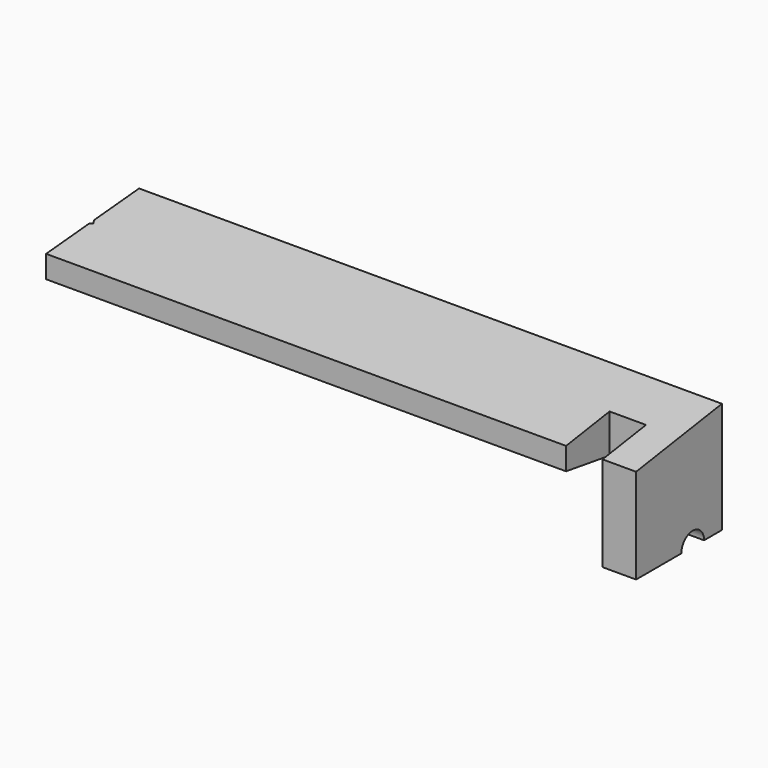
from build123d import *

# Parameters (mm, degrees)
F5_DEPTH  = 69.9135
F7_DEPTH  = 3.98018
F9_DEPTH  = 3.26644
F10_W     = 4.318
F10_H     = 6.4389
F11_DEPTH = 25.4
F12_R     = 1.68275
F13_DEPTH = 69.9145
F16_DEPTH = 13.17344
F18_DEPTH = 13.17344


# Not quite as in the source:
# - a variable given as a bare number and used for a length is read in inches; the dataset says mm whatever the document's units were


with BuildPart() as f5:
    # F4 (on Right) → F5 (new body)
    with BuildSketch(Plane.YZ):
        Polygon((12.7127, 13.17244), (0, 11.24458), (0, 8.59028), (12.7127, 6.66242), align=None)
    extrude(amount=-F5_DEPTH)

    # F6 (on face) → F7 (join)
    with BuildSketch(Plane.YZ):
        Polygon((12.7127, 0), (12.7127, 6.66242), (0, 8.59028), (0, 0), align=None)
    extrude(amount=-F7_DEPTH)

    # F8 (on face) → F9 (join)
    with BuildSketch(Plane(origin=(-3.98018, 0, 0), x_dir=(0, -1, 0), z_dir=(-1, 0, 0))):
        Polygon((-6.4389, 7.6138314286), (-12.7127, 6.66242), (-12.7127, 0), (-6.4389, 0), align=None)
    extrude(amount=F9_DEPTH)

    # F10 (on face) → F11 (cut)
    with BuildSketch(Plane(origin=(0, 0, 0), x_dir=(1, 0, 0), z_dir=(0, 0, -1))):
        with Locations((-6.13918, -3.21945)):
            Rectangle(F10_W, F10_H)
    extrude(amount=-F11_DEPTH, mode=Mode.SUBTRACT)

    # F12 (on face) → F13 (cut, through all)
    with BuildSketch(Plane.YZ):
        with Locations((8.38835, 0)):
            Circle(F12_R)
    extrude(amount=-F13_DEPTH, mode=Mode.SUBTRACT)

    # F15 (on offset) → F16 (cut, through all)
    with BuildSketch(Plane.XY.offset(13.17244)):
        Polygon((-69.9135, 12.7127), (-69.9135, 0), (-69.0626, 12.7127), align=None)
    extrude(amount=-F16_DEPTH, mode=Mode.SUBTRACT)

    # F17 (on offset) → F18 (cut, through all)
    with BuildSketch(Plane.XY.offset(13.17244)):
        Polygon((-69.1999940296, 6.096), (-69.4737402245, 6.570142318), (-69.5177555441, 5.9125403041), align=None)
    extrude(amount=-F18_DEPTH, mode=Mode.SUBTRACT)


solid = f5.part
